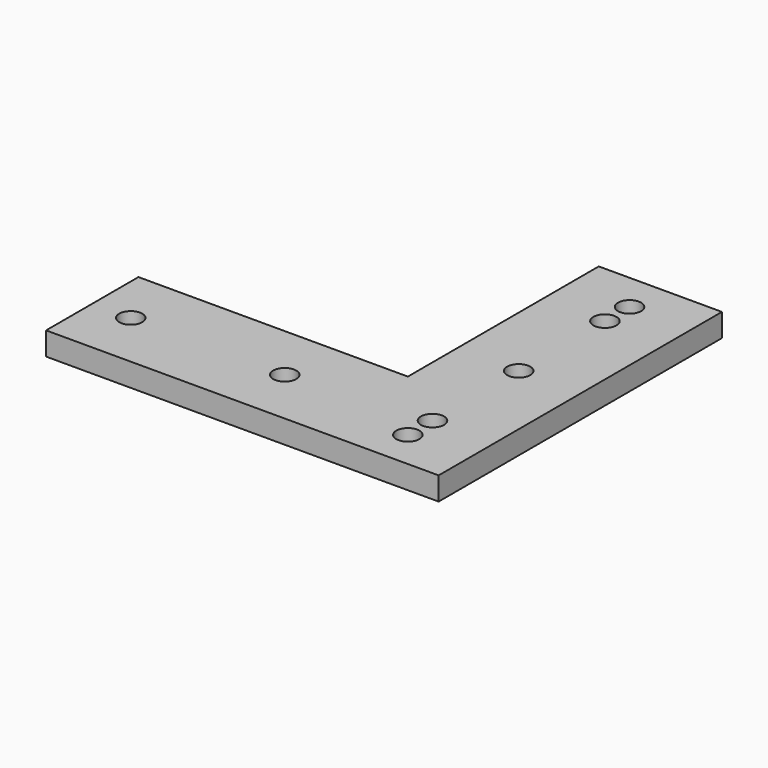
from build123d import *

# Parameters (mm, degrees)
F1_DEPTH = 3
F2_D     = 3


# Not quite as in the source:
# - a feature names something its author has since deleted; it is built from what else it names


with BuildPart() as f1:
    # F0 (on Top) → F1 (new body)
    with BuildSketch(Plane.XY):
        Polygon((0, 31), (0, 0), (-35, 0), (-35, -15), (0, -15), (16, -15), (16, 31), align=None)
    extrude(amount=F1_DEPTH)

    # F2 (through all)
    with Locations(Plane(origin=(0, 0, 0), x_dir=(1, 0, 0), z_dir=(0, 0, -1))):
        with Locations((8, -8), (8, -22), (-10, 7.5), (-30, 7.5), (8, 6), (8, -26), (8, 10)):
            Hole(F2_D / 2)


solid = f1.part
